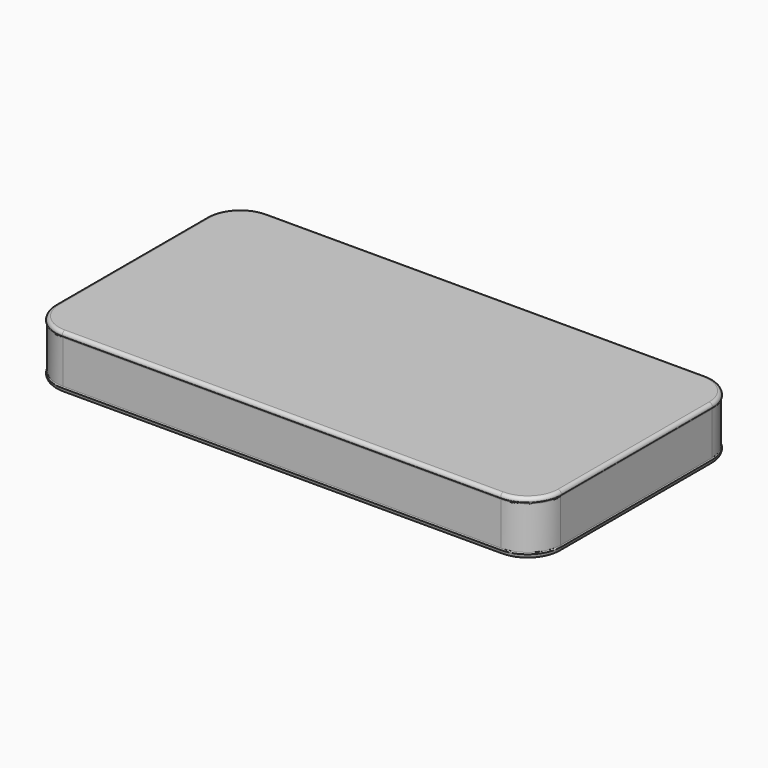
from build123d import *

# Parameters (mm, degrees)
F0_W     = 1905
F0_H     = 965.2
F1_DEPTH = 203.2
F2_R     = 127
F3_R     = 12.7


with BuildPart() as f1:
    # F0 (on Top) → F1 (new body)
    with BuildSketch(Plane.XY):
        Rectangle(F0_W, F0_H)
    extrude(amount=F1_DEPTH)

    # F2
    f2_edges = [f1.edges().sort_by_distance(p)[0] for p in [
        (952.5, -482.6, 101.6),
        (-952.5, -482.6, 101.6),
        (952.5, 482.6, 101.6),
        (-952.5, 482.6, 101.6),
    ]]
    fillet(f2_edges, radius=F2_R)

    # F3
    f3_edges = [f1.edges().sort_by_distance(p)[0] for p in [
        (952.5, 0, 203.2),
        (915.302561, -445.402561, 203.2),
        (915.302561, 445.402561, 203.2),
        (0, -482.6, 203.2),
        (0, 482.6, 203.2),
        (-915.302561, -445.402561, 203.2),
        (-915.302561, 445.402561, 203.2),
        (-952.5, 0, 203.2),
        (952.5, 0, 0),
        (915.302561, -445.402561, 0),
        (915.302561, 445.402561, 0),
        (0, -482.6, 0),
        (0, 482.6, 0),
        (-915.302561, -445.402561, 0),
        (-915.302561, 445.402561, 0),
        (-952.5, 0, 0),
    ]]
    fillet(f3_edges, radius=F3_R)

    # F7: sweep along a path in F7_path
    with BuildLine(Plane(origin=(-825.5, -482.6, 190.5), x_dir=(0, 1, 0), z_dir=(0, 0, 1))) as f7_path:
        Line((0, 0), (0, -1651))
        ThreePointArc((0, -1651), (37.1974387893, -1740.8025612107), (127, -1778))
        Line((127, -1778), (838.2, -1778))
        ThreePointArc((838.2, -1778), (928.0025612107, -1740.8025612107), (965.2, -1651))
        Line((965.2, -1651), (965.2, 0))
        ThreePointArc((965.2, 0), (928.0025612107, 89.8025612107), (838.2, 127))
        Line((838.2, 127), (127, 127))
        ThreePointArc((127, 127), (37.1974387893, 89.8025612107), (0, 0))
    # F5 (on face) → F7 (sweep, cut)
    with BuildSketch(Plane.YZ.offset(825.5)):
        with BuildLine():
            Line((-480.06, 21.058702955), (-480.06, 182.141297045))
            ThreePointArc((-480.06, 182.141297045), (-481.7282889113, 186.4312948633), (-485.8565610336, 188.4671333779))
            Line((-485.8565610336, 188.4671333779), (-553.3473393859, 194.3718113762))
            Line((-553.3473393859, 194.3718113762), (-553.3473393859, 8.8281886238))
            Line((-553.3473393859, 8.8281886238), (-485.8565610336, 14.7328666221))
            ThreePointArc((-485.8565610336, 14.7328666221), (-481.7282889113, 16.7687051367), (-480.06, 21.058702955))
        make_face()
    sweep(path=f7_path.line, mode=Mode.SUBTRACT)


solid = f1.part
